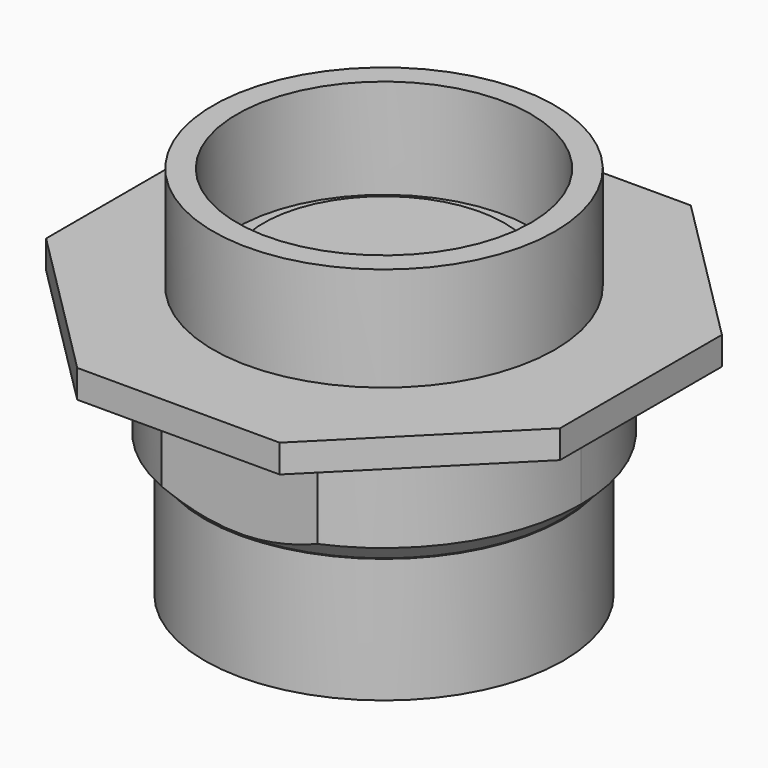
from build123d import *

# Parameters (mm, degrees)
F1_DEPTH    = 2.25
F2_R        = 13.715
F3_DEPTH    = 10.6
F5_DEPTH    = 9.5
F6_T2_ANGLE = 280.2692951884
F6_T4_ANGLE = 100.1752461875
F7_R        = 14.4
F8_DEPTH    = 10
F9_R        = 11.8
F10_DEPTH   = 7
F11_R       = 11.8
F11_R_2     = 9.6734059383
F12_DEPTH   = 8
F13_R       = 9.375
F14_DEPTH   = 1


# Not quite as in the source:
# - a fillet or chamfer that OpenCascade refuses, or shapes differently, is made with other operations: its cross-section is extruded or revolved along the edge and cut away or added


with BuildPart() as f1:
    # F0 (on Top) → F1 (new body)
    with BuildSketch(Plane.XY):
        Polygon((0, 12.5), (12.5, 0), (28.75, 0), (41.25, 12.5), (41.25, 28.75), (28.75, 41.25), (12.5, 41.25), (0, 28.75), align=None)
    extrude(amount=F1_DEPTH)

    # F2 (on Top) → F3 (join)
    with BuildSketch(Plane.XY):
        with Locations((20.625, 20.625)):
            Circle(F2_R)
    extrude(amount=F3_DEPTH)

    # F4 (on face) → F5 (join)
    with BuildSketch(Plane(origin=(0, 0, 0), x_dir=(1, 0, 0), z_dir=(0, 0, -1))):
        with BuildLine():
            ThreePointArc((14.3488546862, -6.125), (11.9509898535, -33.8311178239), (36.425, -20.625))
            ThreePointArc((36.425, -20.625), (33.8311178239, -11.9509898535), (26.9011453138, -6.125))
            Line((26.9011453138, -6.125), (14.3488546862, -6.125))
        make_face()
    extrude(amount=F5_DEPTH)

    # F6: chamfer of 1.5 on 2 edges, made by hand

    # F6_s1 → F6_t2 (revolve, cut)
    with BuildSketch(Plane(origin=(23.5875160096, 4.2735214072, 0), x_dir=(0, 0, 1), z_dir=(0.9839807168, 0.1782749254, 0))):
        with BuildLine():
            Line((-7.9575735931, -0.7752555397), (-9.5424264069, -2.3601083535))
            Line((-9.5424264069, -2.3601083535), (-9.5724264069, -2.3601083535))
            ThreePointArc((-9.5724264069, -2.3601083535), (-9.53, -1.58889515), (-9.53, -0.8176819466))
            Line((-9.53, -0.8176819466), (-9.5, -0.7876819466))
            ThreePointArc((-9.5, -0.7876819466), (-8.7287867966, -0.7876819466), (-7.9575735931, -0.7452555397))
            Line((-7.9575735931, -0.7452555397), (-7.9575735931, -0.7752555397))
        make_face()
    revolve(axis=Axis((20.625, 20.625, -9.5), (0, 0, -1)), revolution_arc=F6_T2_ANGLE, mode=Mode.SUBTRACT)

    # F6_s3 → F6_t4 (revolve, cut)
    with BuildSketch(Plane.XZ.offset(-20.625)):
        with BuildLine():
            Line((36.4674264069, -7.9575735931), (34.8825735931, -9.5424264069))
            Line((34.8825735931, -9.5424264069), (34.8825735931, -9.5724264069))
            ThreePointArc((34.8825735931, -9.5724264069), (35.6537867966, -9.53), (36.425, -9.53))
            Line((36.425, -9.53), (36.455, -9.5))
            ThreePointArc((36.455, -9.5), (36.455, -8.7287867966), (36.4974264069, -7.9575735931))
            Line((36.4974264069, -7.9575735931), (36.4674264069, -7.9575735931))
        make_face()
    revolve(axis=Axis((20.625, 20.625, -9.5), (0, 0, -1)), revolution_arc=F6_T4_ANGLE, mode=Mode.SUBTRACT)

    # F7 (on face) → F8 (join)
    with BuildSketch(Plane(origin=(0, 0, -9.5), x_dir=(1, 0, 0), z_dir=(0, 0, -1))):
        with Locations((20.625, -20.625)):
            Circle(F7_R)
    extrude(amount=F8_DEPTH)

    # F9 (on face) → F10 (cut)
    with BuildSketch(Plane.XY.offset(10.6)):
        with Locations((20.625, 20.625)):
            Circle(F9_R)
    extrude(amount=-F10_DEPTH, mode=Mode.SUBTRACT)

    # F11 (on face) → F12 (cut)
    with BuildSketch(Plane.XY.offset(10.6)):
        with Locations((20.625, 20.625)):
            Circle(F11_R)
        with Locations((20.625, 20.625)):
            Circle(F11_R_2, mode=Mode.SUBTRACT)
    extrude(amount=-F12_DEPTH, mode=Mode.SUBTRACT)

    # F13 (on face) → F14 (cut)
    with BuildSketch(Plane(origin=(0, 0, -19.5), x_dir=(1, 0, 0), z_dir=(0, 0, -1))):
        with Locations((20.625, -20.625)):
            Circle(F13_R)
    extrude(amount=-F14_DEPTH, mode=Mode.SUBTRACT)


solid = f1.part
